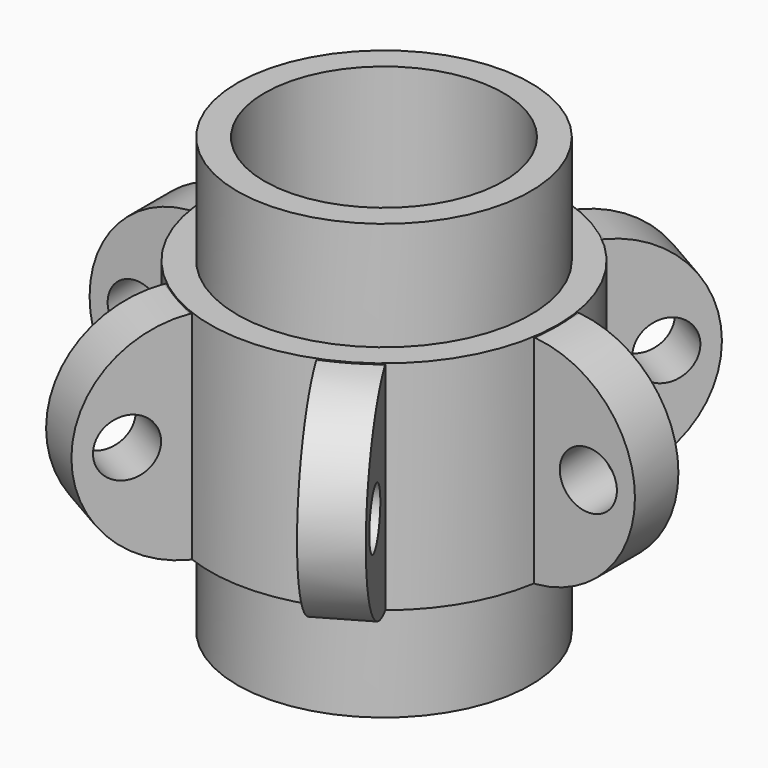
from build123d import *

# Parameters (mm, degrees)
F0_W            = 12.7
F0_H            = 50.8
F2_W            = 5.08
F2_H            = 50.5912028922
F3_DEPTH        = 6.35
F3_DEPTH_BACK   = 6.35
F3_COPIES_COUNT = 6
F4_R            = 6.6777820133
F5_DEPTH        = 25.4
F5_COPIES_COUNT = 6
F7_W            = 6.35
F7_H            = 101.6


# Not quite as in the source:
# - a pattern or mirror of a feature is missing from the dataset's text; its kind, count and spacing are read off the source's solid


with BuildPart() as f1:
    # F0 (on Front) → F1 (revolve)
    with BuildSketch(Plane.XZ):
        with Locations((-34.29, 25.4)):
            Rectangle(F0_W, F0_H)
    revolve(axis=Axis((0, 0, 19.3039998412), (0, 0, 1)))

    # F2 (on Front) → F3 (join, two sides)
    with BuildSketch(Plane.XZ) as f3_sk:
        with BuildLine():
            Line((-40.64, 0), (-40.64, 50.5912028922))
            ThreePointArc((-40.64, 50.5912028922), (-63.7394462668, 25.2956014461), (-40.64, 0))
        make_face()
        with Locations((-38.1, 25.2956014461)):
            Rectangle(F2_W, F2_H)
    f3 = extrude(amount=F3_DEPTH) + extrude(f3_sk.sketch, amount=-F3_DEPTH_BACK)

    # F3_copies: F3 ×6 about axis
    f3_copies_axis = Axis((0, 0, 0), (0, 0, 1))
    for i in range(1, F3_COPIES_COUNT):
        add(f3.rotate(f3_copies_axis, i * 360 / F3_COPIES_COUNT))

    # F4 (on face) → F5 (cut)
    with BuildSketch(Plane.XZ.offset(6.35)):
        with Locations((-52.8408407984, 25.4)):
            Circle(F4_R)
    f5 = extrude(amount=-F5_DEPTH, mode=Mode.SUBTRACT)

    # F5_copies: F5 ×6 about axis
    f5_copies_axis = Axis((0, 0, 0), (0, 0, 1))
    for i in range(1, F5_COPIES_COUNT):
        add(f5.rotate(f5_copies_axis, i * 360 / F5_COPIES_COUNT), mode=Mode.SUBTRACT)

    # F7 (on Front) → F8 (revolve)
    with BuildSketch(Plane.XZ):
        with Locations((-31.115, 25.4)):
            Rectangle(F7_W, F7_H)
    revolve(axis=Axis((0, 0, 73.8201290369), (0, 0, 1)))


solid = f1.part
